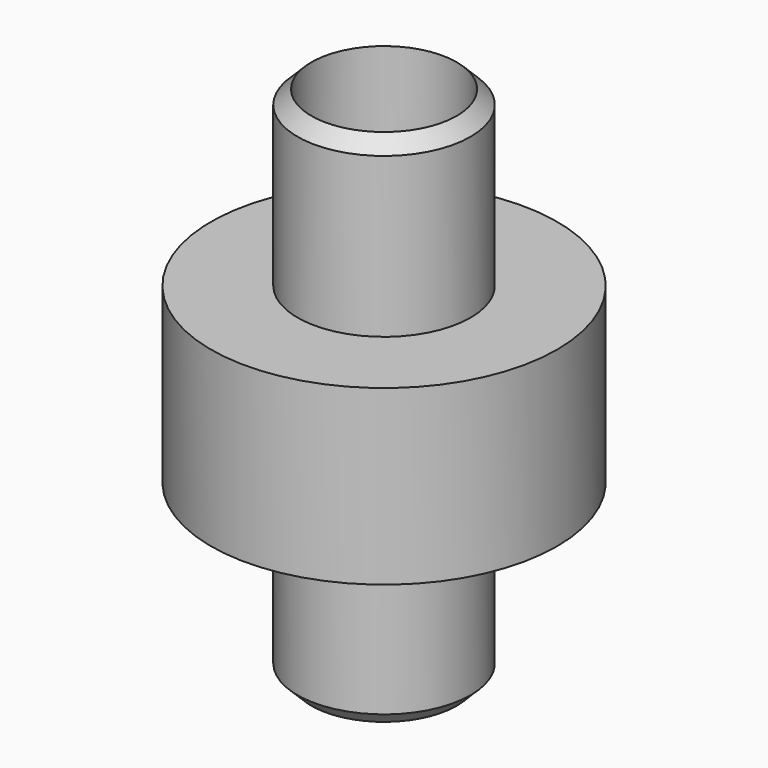
from build123d import *

# Parameters (mm, degrees)
F0_R      = 1.5875
F1_DEPTH  = 3.175
F2_R      = 3.175
F3_DEPTH  = 3.175
F4_R      = 1.5875
F5_DEPTH  = 3.175
F6_T      = -0.254
F7_DEPTH  = 0.254
F8_SIZE   = 0.25399
F10_DEPTH = 4.175


# Not quite as in the source:
# - a fillet or chamfer is up to 0.001 mm smaller than in the source, because OpenCascade refuses the exact size


with BuildPart() as f1:
    # F0 (on Top) → F1 (new body)
    with BuildSketch(Plane.XY):
        Circle(F0_R)
    extrude(amount=F1_DEPTH)

    # F2 (on face) → F3 (join)
    with BuildSketch(Plane.XY.offset(3.175)):
        Circle(F2_R)
    extrude(amount=F3_DEPTH)

    # F4 (on face) → F5 (join)
    with BuildSketch(Plane.XY.offset(6.35)):
        Circle(F4_R)
    extrude(amount=F5_DEPTH)

    # F6
    f6_openings = [f1.faces().sort_by_distance(p)[0] for p in [
        (0, 0, 9.525),
    ]]
    offset(amount=F6_T, openings=f6_openings, kind=Kind.INTERSECTION)

    # F7 (cut, through all): a face of the model
    f7_faces = [f1.faces().sort_by_distance(p)[0] for p in [
        (0, 0, 0.254),
    ]]
    extrude(f7_faces, amount=-F7_DEPTH, mode=Mode.SUBTRACT)

    # F8 (size 0.254 in the source; OpenCascade refuses exactly that, so slightly less here)
    f8_edges = [f1.edges().sort_by_distance(p)[0] for p in [
        (-1.5875, 0, 9.525),
        (-1.5875, 0, 0),
    ]]
    chamfer(f8_edges, length=F8_SIZE)

    # F9 (on Front) → F10 (cut, up to face)
    with BuildSketch(Plane.XZ):
        Polygon((1.0448596497, 5.36575), (-1.0448596497, 5.36575), (0, 3.556), align=None)
    extrude(amount=-F10_DEPTH, mode=Mode.SUBTRACT)


solid = f1.part
